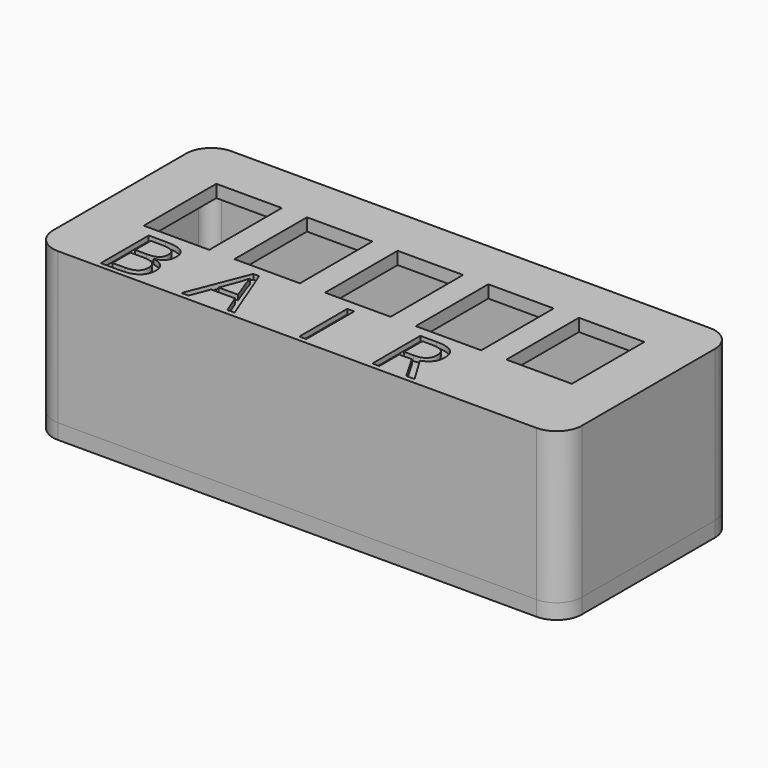
from build123d import *

# Parameters (mm, degrees)
F0_W         = 105
F0_H         = 43
F0_W_2       = 13
F0_H_2       = 18
F1_DEPTH     = 30
F2_R         = 5
F3_T         = -2.5
F4_DEPTH     = 30
F5_TEXT_SIZE = 16.6666666667
F6_DEPTH     = 1
F8_DEPTH     = 3
F9_DEPTH     = 3


# Not quite as in the source:
# - Text() gives the source's letters only with a copy of the font that has no kerning and outlines rounded to 1/6400 em; it was checked with that copy


with BuildPart() as f1:
    # F0 (on Top) → F1 (new body)
    with BuildSketch(Plane.XY):
        with Locations((0, 21.5)):
            Rectangle(F0_W, F0_H)
        with Locations((-36, 24)):
            Rectangle(F0_W_2, F0_H_2, mode=Mode.SUBTRACT)
        with Locations((-18, 24)):
            Rectangle(F0_W_2, F0_H_2, mode=Mode.SUBTRACT)
        with Locations((0, 24)):
            Rectangle(F0_W_2, F0_H_2, mode=Mode.SUBTRACT)
        with Locations((18, 24)):
            Rectangle(F0_W_2, F0_H_2, mode=Mode.SUBTRACT)
        with Locations((36, 24)):
            Rectangle(F0_W_2, F0_H_2, mode=Mode.SUBTRACT)
        with Locations((-36, 24)):
            Rectangle(F0_W_2, F0_H_2)
        with Locations((-18, 24)):
            Rectangle(F0_W_2, F0_H_2)
        with Locations((0, 24)):
            Rectangle(F0_W_2, F0_H_2)
        with Locations((18, 24)):
            Rectangle(F0_W_2, F0_H_2)
        with Locations((36, 24)):
            Rectangle(F0_W_2, F0_H_2)
    extrude(amount=F1_DEPTH)

    # F2
    f2_edges = [f1.edges().sort_by_distance(p)[0] for p in [
        (-52.5, 0, 15),
        (52.5, 0, 15),
        (52.5, 43, 15),
        (-52.5, 43, 15),
    ]]
    fillet(f2_edges, radius=F2_R)

    # F3
    f3_openings = [f1.faces().sort_by_distance(p)[0] for p in [
        (0, 21.5, 0),
    ]]
    offset(amount=F3_T, openings=f3_openings)

    # F0 (on Top) → F4 (cut, through all)
    with BuildSketch(Plane.XY):
        with Locations((-36, 24)):
            Rectangle(F0_W_2, F0_H_2)
        with Locations((-18, 24)):
            Rectangle(F0_W_2, F0_H_2)
        with Locations((0, 24)):
            Rectangle(F0_W_2, F0_H_2)
        with Locations((18, 24)):
            Rectangle(F0_W_2, F0_H_2)
        with Locations((36, 24)):
            Rectangle(F0_W_2, F0_H_2)
    extrude(amount=F4_DEPTH, mode=Mode.SUBTRACT)

    # F5 (on face) → F6 (cut)
    with BuildSketch(Plane.XY.offset(30)):
        with Locations((-41.48046875, 1)):
            Text('B', F5_TEXT_SIZE, font='Open Sans', text_align=(TextAlign.LEFT, TextAlign.BOTTOM))
        with Locations((-23.8138020833, 1)):
            Text('A', F5_TEXT_SIZE, font='Open Sans', text_align=(TextAlign.LEFT, TextAlign.BOTTOM))
        with Locations((-2.0494791667, 1)):
            Text('I', F5_TEXT_SIZE, font='Open Sans', text_align=(TextAlign.LEFT, TextAlign.BOTTOM))
        with Locations((12.4505208333, 1)):
            Text('R', F5_TEXT_SIZE, font='Open Sans', text_align=(TextAlign.LEFT, TextAlign.BOTTOM))
    extrude(amount=-F6_DEPTH, mode=Mode.SUBTRACT)


with BuildPart() as f8:
    # F7 (on face) → F8 (new body)
    with BuildSketch(Plane(origin=(0, 0, 0), x_dir=(1, 0, 0), z_dir=(0, 0, -1))):
        with BuildLine():
            ThreePointArc((-52.5, -38), (-51.0355339059, -41.5355339059), (-47.5, -43))
            Line((-47.5, -43), (47.5, -43))
            ThreePointArc((47.5, -43), (51.0355339059, -41.5355339059), (52.5, -38))
            Line((52.5, -38), (52.5, -5))
            ThreePointArc((52.5, -5), (51.0355339059, -1.4644660941), (47.5, 0))
            Line((47.5, 0), (-47.5, 0))
            ThreePointArc((-47.5, 0), (-51.0355339059, -1.4644660941), (-52.5, -5))
            Line((-52.5, -5), (-52.5, -38))
        make_face()
        with BuildLine():
            ThreePointArc((-50, -5), (-49.267766953, -3.232233047), (-47.5, -2.5))
            Line((-47.5, -2.5), (47.5, -2.5))
            ThreePointArc((47.5, -2.5), (49.267766953, -3.232233047), (50, -5))
            Line((50, -5), (50, -38))
            ThreePointArc((50, -38), (49.267766953, -39.767766953), (47.5, -40.5))
            Line((47.5, -40.5), (-47.5, -40.5))
            ThreePointArc((-47.5, -40.5), (-49.267766953, -39.767766953), (-50, -38))
            Line((-50, -38), (-50, -5))
        make_face(mode=Mode.SUBTRACT)
        with BuildLine():
            Line((47.5, -2.5), (-47.5, -2.5))
            ThreePointArc((-47.5, -2.5), (-49.267766953, -3.232233047), (-50, -5))
            Line((-50, -5), (-50, -38))
            ThreePointArc((-50, -38), (-49.267766953, -39.767766953), (-47.5, -40.5))
            Line((-47.5, -40.5), (47.5, -40.5))
            ThreePointArc((47.5, -40.5), (49.267766953, -39.767766953), (50, -38))
            Line((50, -38), (50, -5))
            ThreePointArc((50, -5), (49.267766953, -3.232233047), (47.5, -2.5))
        make_face()
        with BuildLine():
            ThreePointArc((47.5, -36), (46.9142135624, -37.4142135624), (45.5, -38))
            Line((45.5, -38), (-45.5, -38))
            ThreePointArc((-45.5, -38), (-46.9142135624, -37.4142135624), (-47.5, -36))
            Line((-47.5, -36), (-47.5, -7))
            ThreePointArc((-47.5, -7), (-46.9142135624, -5.5857864376), (-45.5, -5))
            Line((-45.5, -5), (45.5, -5))
            ThreePointArc((45.5, -5), (46.9142135624, -5.5857864376), (47.5, -7))
            Line((47.5, -7), (47.5, -36))
        make_face(mode=Mode.SUBTRACT)
        with BuildLine():
            Line((-45.5, -38), (45.5, -38))
            ThreePointArc((45.5, -38), (46.9142135624, -37.4142135624), (47.5, -36))
            Line((47.5, -36), (47.5, -7))
            ThreePointArc((47.5, -7), (46.9142135624, -5.5857864376), (45.5, -5))
            Line((45.5, -5), (-45.5, -5))
            ThreePointArc((-45.5, -5), (-46.9142135624, -5.5857864376), (-47.5, -7))
            Line((-47.5, -7), (-47.5, -36))
            ThreePointArc((-47.5, -36), (-46.9142135624, -37.4142135624), (-45.5, -38))
        make_face()
    extrude(amount=F8_DEPTH)

    # F7 (on face) → F9 (join)
    with BuildSketch(Plane(origin=(0, 0, 0), x_dir=(1, 0, 0), z_dir=(0, 0, -1))):
        with BuildLine():
            Line((47.5, -2.5), (-47.5, -2.5))
            ThreePointArc((-47.5, -2.5), (-49.267766953, -3.232233047), (-50, -5))
            Line((-50, -5), (-50, -38))
            ThreePointArc((-50, -38), (-49.267766953, -39.767766953), (-47.5, -40.5))
            Line((-47.5, -40.5), (47.5, -40.5))
            ThreePointArc((47.5, -40.5), (49.267766953, -39.767766953), (50, -38))
            Line((50, -38), (50, -5))
            ThreePointArc((50, -5), (49.267766953, -3.232233047), (47.5, -2.5))
        make_face()
        with BuildLine():
            ThreePointArc((47.5, -36), (46.9142135624, -37.4142135624), (45.5, -38))
            Line((45.5, -38), (-45.5, -38))
            ThreePointArc((-45.5, -38), (-46.9142135624, -37.4142135624), (-47.5, -36))
            Line((-47.5, -36), (-47.5, -7))
            ThreePointArc((-47.5, -7), (-46.9142135624, -5.5857864376), (-45.5, -5))
            Line((-45.5, -5), (45.5, -5))
            ThreePointArc((45.5, -5), (46.9142135624, -5.5857864376), (47.5, -7))
            Line((47.5, -7), (47.5, -36))
        make_face(mode=Mode.SUBTRACT)
    extrude(amount=-F9_DEPTH)


solid = Compound([f1.part, f8.part])
